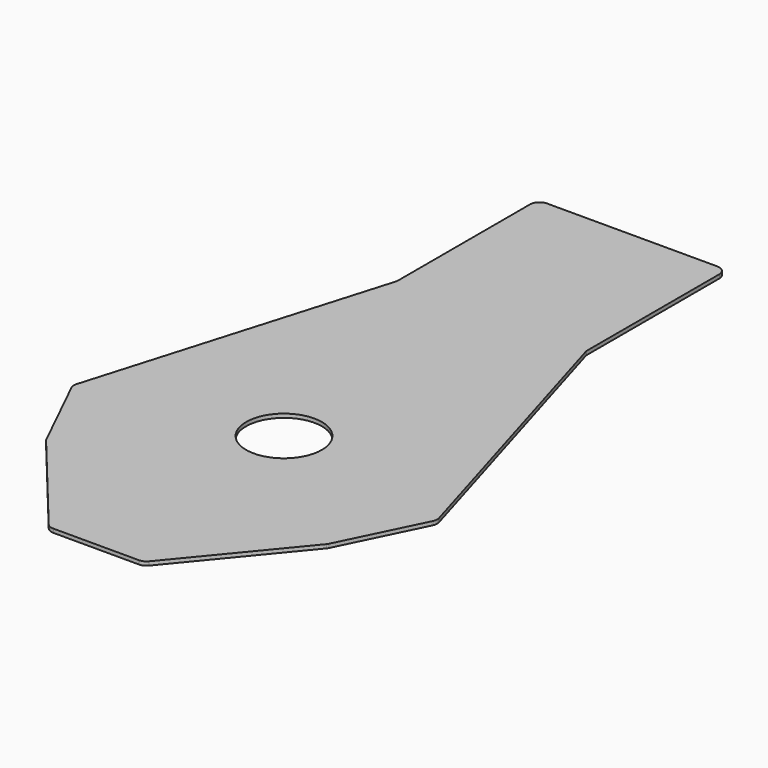
from build123d import *

# Parameters (mm, degrees)
F1_R     = 20
F1_W     = 2
F1_H     = 20
F1_R_2   = 10
F2_DEPTH = 2
F3_R     = 5
F5_D     = 3.3
F6_R     = 20
F7_DEPTH = 2
F8_R     = 5


with BuildPart() as f2:
    # F1 (on Top) → F2 (new body)
    with BuildSketch(Plane.XY):
        Polygon((-74.397836401, -64.1479690937), (-25, -124.0796787573), (25, -124.0796787573), (74.397836401, -64.1479690937), (96.336236162, -19.2179499982), (22.5, 230), (-22.5, 230), (-96.336236162, -19.2179499982), align=None)
        with BuildLine():
            Line((-24.5530502594, -108.8994547314), (-60.4716474798, -65.321373241))
            ThreePointArc((-60.4716474798, -65.321373241), (-61.4996911033, -61.081257714), (-58.8071732987, -57.6482122372))
            Line((-58.8071732987, -57.6482122372), (-12.0794250934, -34.8320185054))
            ThreePointArc((-12.0794250934, -34.8320185054), (-6.8077487763, -35.3845986788), (-4.9950577161, -40.3655691827))
            Line((-4.9950577161, -40.3655691827), (-19.3037453244, -107.6156885355))
            ThreePointArc((-19.3037453244, -107.6156885355), (-21.5253867426, -109.9054790926), (-24.5530502594, -108.8994547314))
        make_face(mode=Mode.SUBTRACT)
        Polygon((-59.7563114694, -2.9695777864), (-44.1362007471, 9.5209042308), (-42.8871525454, 7.9588931586), (-58.5072632677, -4.5315888586), align=None, mode=Mode.SUBTRACT)
        Polygon((-11.6469311007, 32.9398571929), (-27.267041823, 20.4493751757), (-28.5160900247, 22.011386248), (-12.8959793024, 34.5018682652), align=None, mode=Mode.SUBTRACT)
        with BuildLine():
            Line((-11.7288579458, -110.4553494967), (-2.9343164407, -69.1214422886))
            ThreePointArc((-2.9343164407, -69.1214422886), (0, -66.7457715493), (2.9343164407, -69.1214422886))
            Line((2.9343164407, -69.1214422886), (11.7288579458, -110.4553494967))
            ThreePointArc((11.7288579458, -110.4553494967), (11.126170526, -112.9674038721), (8.7945415051, -114.0796787573))
            Line((8.7945415051, -114.0796787573), (-8.7945415051, -114.0796787573))
            ThreePointArc((-8.7945415051, -114.0796787573), (-11.126170526, -112.9674038721), (-11.7288579458, -110.4553494967))
        make_face(mode=Mode.SUBTRACT)
        with BuildLine():
            ThreePointArc((58.8071732987, -57.6482122372), (61.4996911033, -61.081257714), (60.4716474798, -65.321373241))
            Line((60.4716474798, -65.321373241), (24.5530502594, -108.8994547314))
            ThreePointArc((24.5530502594, -108.8994547314), (21.5253867426, -109.9054790926), (19.3037453244, -107.6156885355))
            Line((19.3037453244, -107.6156885355), (4.9950577161, -40.3655691827))
            ThreePointArc((4.9950577161, -40.3655691827), (6.8077487763, -35.3845986788), (12.0794250934, -34.8320185054))
            Line((12.0794250934, -34.8320185054), (58.8071732987, -57.6482122372))
        make_face(mode=Mode.SUBTRACT)
        Circle(F1_R, mode=Mode.SUBTRACT)
        Polygon((11.6469311007, 32.9398571929), (12.8959793024, 34.5018682652), (28.5160900247, 22.011386248), (27.267041823, 20.4493751757), align=None, mode=Mode.SUBTRACT)
        with Locations((0, 35)):
            Rectangle(F1_W, F1_H, mode=Mode.SUBTRACT)
        Polygon((44.1362007471, 9.5209042308), (59.7563114694, -2.9695777864), (58.5072632677, -4.5315888586), (42.8871525454, 7.9588931586), align=None, mode=Mode.SUBTRACT)
        with BuildLine():
            Line((-67.0381035794, 9.2654395509), (-19.7940226257, 168.7274275506))
            ThreePointArc((-19.7940226257, 168.7274275506), (-14.2824044066, 172.2553318396), (-10, 167.3070941165))
            Line((-10, 167.3070941165), (-10, 45.6234134578))
            ThreePointArc((-10, 45.6234134578), (-10.4937209074, 43.4569765814), (-11.8773794957, 41.7183857772))
            Line((-11.8773794957, 41.7183857772), (-59.1214604493, 3.9400784362))
            ThreePointArc((-59.1214604493, 3.9400784362), (-65.0348270928, 3.6964031886), (-67.0381035794, 9.2654395509))
        make_face(mode=Mode.SUBTRACT)
        with Locations((0, 75)):
            Rectangle(F1_W, F1_H, mode=Mode.SUBTRACT)
        with BuildLine():
            ThreePointArc((11.8773794957, 41.7183857772), (10.4937209074, 43.4569765814), (10, 45.6234134578))
            Line((10, 45.6234134578), (10, 167.3070941165))
            ThreePointArc((10, 167.3070941165), (14.2824044066, 172.2553318396), (19.7940226257, 168.7274275506))
            Line((19.7940226257, 168.7274275506), (67.0381035794, 9.2654395509))
            ThreePointArc((67.0381035794, 9.2654395509), (65.0348270928, 3.6964031886), (59.1214604493, 3.9400784362))
            Line((59.1214604493, 3.9400784362), (11.8773794957, 41.7183857772))
        make_face(mode=Mode.SUBTRACT)
        with Locations((0, 115)):
            Rectangle(F1_W, F1_H, mode=Mode.SUBTRACT)
        with Locations((0, 155)):
            Rectangle(F1_W, F1_H, mode=Mode.SUBTRACT)
        with Locations((0, 205)):
            Circle(F1_R_2, mode=Mode.SUBTRACT)
    extrude(amount=F2_DEPTH)

    # F3
    f3_edges = [f2.edges().sort_by_distance(p)[0] for p in [
        (-25, -124.079679, 1),
        (25, -124.079679, 1),
        (-74.397836, -64.147969, 1),
        (-96.336236, -19.21795, 1),
        (74.397836, -64.147969, 1),
        (96.336236, -19.21795, 1),
        (22.5, 230, 1),
        (-22.5, 230, 1),
    ]]
    fillet(f3_edges, radius=F3_R)

    # F5 (through all)
    with Locations(Plane.XY.offset(2)):
        with Locations((-16, 185), (16, 185), (0, 185), (16, 225), (-16, 225), (-87.8943222955, -25.1115134593), (-73.8537464484, -53.8667256804), (-20, -119.0796787573), (20, -119.0796787573), (73.8537464484, -53.8667256804), (87.8943222955, -25.1115134593)):
            Hole(F5_D / 2)


with BuildPart() as f7:
    # F6 (on Top) → F7 (new body)
    with BuildSketch(Plane.XY):
        Polygon((-96.336236162, -19.2179499982), (-74.397836401, -64.1479690937), (-25, -124.0796787573), (25, -124.0796787573), (74.397836401, -64.1479690937), (96.336236162, -19.2179499982), (50, 136.3694951899), (50, 230), (-50, 230), (-50, 136.3694951899), align=None)
        Circle(F6_R, mode=Mode.SUBTRACT)
    extrude(amount=F7_DEPTH)

    # F8
    f8_edges = [f7.edges().sort_by_distance(p)[0] for p in [
        (25, -124.079679, 1),
        (-25, -124.079679, 1),
        (74.397836, -64.147969, 1),
        (96.336236, -19.21795, 1),
        (-74.397836, -64.147969, 1),
        (-96.336236, -19.21795, 1),
        (-50, 136.369495, 1),
        (50, 136.369495, 1),
        (50, 230, 1),
        (-50, 230, 1),
    ]]
    fillet(f8_edges, radius=F8_R)


solid = Compound([f2.part, f7.part])
